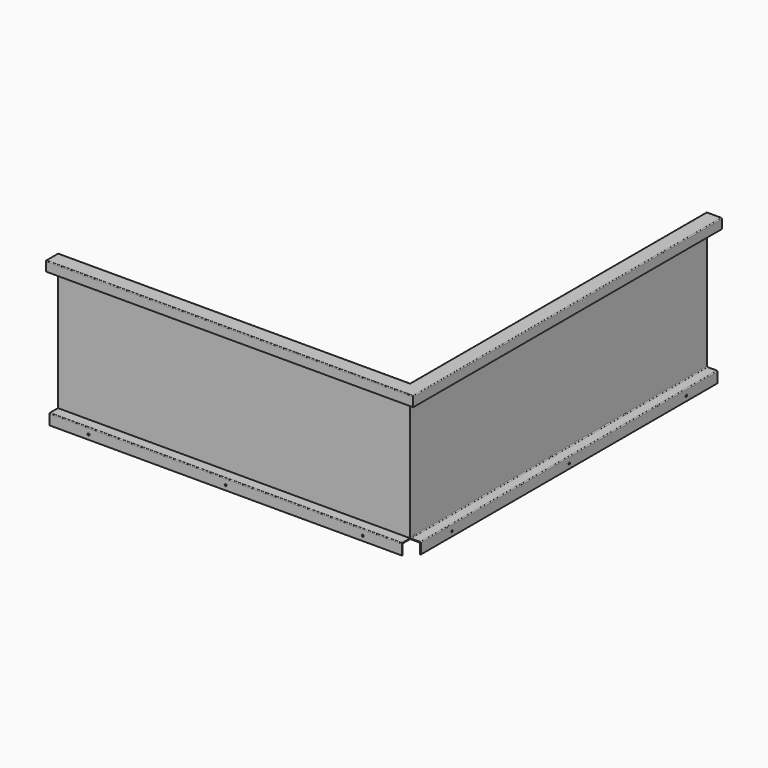
from build123d import *

# Parameters (mm, degrees)
F3_W         = 27
F3_H         = 27
F4_DEPTH     = 30
F5_T1_DEPTH  = 950
F5_T3_DEPTH  = 986
F5_T5_DEPTH  = 902
F5_T7_DEPTH  = 938
F5_T13_DEPTH = 955
F5_T17_DEPTH = 907
F5_T20_DEPTH = 960
F5_T22_DEPTH = 998
F5_T24_DEPTH = 953
F5_T26_DEPTH = 950
F5_T28_DEPTH = 905
F5_T30_DEPTH = 912
F5_T36_DEPTH = 910
F5_T40_DEPTH = 958
F5_T47_DEPTH = 910
F5_T51_DEPTH = 958
F8_D         = 5
F8_ON_F6_D   = 5


# Not quite as in the source:
# - a fillet or chamfer that OpenCascade refuses, or shapes differently, is made with other operations: its cross-section is extruded or revolved along the edge and cut away or added


with BuildPart() as f2:
    # F2: sweep along a path in F1
    with BuildLine(Plane.XY) as f2_path:
        Line((0, 0), (0, -948))
        Line((0, -948), (-900, -948))
    # F0 (on Front) → F2 (sweep)
    with BuildSketch(Plane.XZ):
        Polygon((38, -2), (38, -25), (40, -25), (40, 0), (0, 0), (0, -350), (27, -350), (27, -376), (29, -376), (29, -348), (2, -348), (2, -2), align=None)
    sweep(path=f2_path.line, transition=Transition.RIGHT)

    # F3 (on face) → F4 (cut)
    with BuildSketch(Plane.XY.offset(-348)):
        with Locations((15.5, -963.5)):
            Rectangle(F3_W, F3_H)
    extrude(amount=-F4_DEPTH, mode=Mode.SUBTRACT)

    # F5: fillet of radius 2 on 15 edges, made by hand

    # F5_s2 → F5_t1 (join)
    with BuildSketch(Plane.XZ):
        with BuildLine():
            ThreePointArc((2, -346), (2.5857864376, -347.4142135624), (4, -348))
            Line((4, -348), (2, -348))
            Line((2, -348), (2, -346))
        make_face()
        with BuildLine():
            ThreePointArc((25, -350), (26.4142135624, -350.5857864376), (27, -352))
            Line((27, -352), (27, -350))
            Line((27, -350), (25, -350))
        make_face()
        with BuildLine():
            ThreePointArc((4, -2), (2.5857864376, -2.5857864376), (2, -4))
            Line((2, -4), (2, -2))
            Line((2, -2), (4, -2))
        make_face()
    extrude(amount=F5_T1_DEPTH)

    # F5_s4 → F5_t3 (join)
    with BuildSketch(Plane.XZ):
        with BuildLine():
            ThreePointArc((38, -4), (37.4142135624, -2.5857864376), (36, -2))
            Line((36, -2), (38, -2))
            Line((38, -2), (38, -4))
        make_face()
    extrude(amount=F5_T3_DEPTH)

    # F5_s6 → F5_t5 (join)
    with BuildSketch(Plane.YZ.offset(-900)):
        with BuildLine():
            ThreePointArc((-973, -350), (-974.4142135624, -350.5857864376), (-975, -352))
            Line((-975, -352), (-975, -350))
            Line((-975, -350), (-973, -350))
        make_face()
        with BuildLine():
            ThreePointArc((-952, -2), (-950.5857864376, -2.5857864376), (-950, -4))
            Line((-950, -4), (-950, -2))
            Line((-950, -2), (-952, -2))
        make_face()
    extrude(amount=F5_T5_DEPTH)

    # F5_s8 → F5_t7 (join)
    with BuildSketch(Plane.YZ.offset(-900)):
        with BuildLine():
            ThreePointArc((-984, -2), (-985.4142135624, -2.5857864376), (-986, -4))
            Line((-986, -4), (-986, -2))
            Line((-986, -2), (-984, -2))
        make_face()
    extrude(amount=F5_T7_DEPTH)


with BuildPart() as f5_tool11:
    # F5_s12 → F5_t13 (new body)
    with BuildSketch(Plane.XZ):
        with BuildLine():
            ThreePointArc((4, -2), (2.5857864376, -2.5857864376), (2, -4))
            Line((2, -4), (2, -2))
            Line((2, -2), (4, -2))
        make_face()
    extrude(amount=F5_T13_DEPTH)

    split(bisect_by=Plane.XZ.offset(950), keep=Keep.TOP)


with BuildPart() as f5_tool15:
    # F5_s16 → F5_t17 (new body)
    with BuildSketch(Plane.YZ.offset(7)):
        with BuildLine():
            ThreePointArc((-952, -2), (-950.5857864376, -2.5857864376), (-950, -4))
            Line((-950, -4), (-950, -2))
            Line((-950, -2), (-952, -2))
        make_face()
    extrude(amount=-F5_T17_DEPTH)

    split(bisect_by=Plane.YZ.offset(2), keep=Keep.TOP)


with BuildPart() as f5_tool11_1:
    add(f5_tool11.part)

    # F5_t19: intersect F5_tool15
    add(f5_tool15.part, mode=Mode.INTERSECT)


with BuildPart() as f2_1:
    add(f2.part)

    # F5_t9: union F5_tool11
    add(f5_tool11_1.part)

    # F5_s21 → F5_t20 (cut)
    with BuildSketch(Plane.XZ.offset(-5)):
        with BuildLine():
            ThreePointArc((27, -348), (28.4142135624, -348.5857864376), (29, -350))
            Line((29, -350), (29, -348))
            Line((29, -348), (27, -348))
        make_face()
    extrude(amount=F5_T20_DEPTH, mode=Mode.SUBTRACT)

    # F5_s23 → F5_t22 (cut)
    with BuildSketch(Plane.XZ.offset(-5)):
        with BuildLine():
            ThreePointArc((38, 0), (39.4142135624, -0.5857864376), (40, -2))
            Line((40, -2), (40, 0))
            Line((40, 0), (38, 0))
        make_face()
    extrude(amount=F5_T22_DEPTH, mode=Mode.SUBTRACT)

    # F5_s25 → F5_t24 (cut)
    with BuildSketch(Plane.XZ.offset(-5)):
        with BuildLine():
            ThreePointArc((0, -2), (0.5857864376, -0.5857864376), (2, 0))
            Line((2, 0), (0, 0))
            Line((0, 0), (0, -2))
        make_face()
        with BuildLine():
            ThreePointArc((2, -350), (0.5857864376, -349.4142135624), (0, -348))
            Line((0, -348), (0, -350))
            Line((0, -350), (2, -350))
        make_face()
    extrude(amount=F5_T24_DEPTH, mode=Mode.SUBTRACT)

    # F5_s27 → F5_t26 (cut)
    with BuildSketch(Plane.YZ.offset(-905)):
        with BuildLine():
            ThreePointArc((-988, -2), (-987.4142135624, -0.5857864376), (-986, 0))
            Line((-986, 0), (-988, 0))
            Line((-988, 0), (-988, -2))
        make_face()
    extrude(amount=F5_T26_DEPTH, mode=Mode.SUBTRACT)

    # F5_s29 → F5_t28 (cut)
    with BuildSketch(Plane.YZ.offset(-905)):
        with BuildLine():
            ThreePointArc((-948, -2), (-948.5857864376, -0.5857864376), (-950, 0))
            Line((-950, 0), (-948, 0))
            Line((-948, 0), (-948, -2))
        make_face()
        with BuildLine():
            ThreePointArc((-948, -348), (-948.5857864376, -349.4142135624), (-950, -350))
            Line((-950, -350), (-948, -350))
            Line((-948, -350), (-948, -348))
        make_face()
    extrude(amount=F5_T28_DEPTH, mode=Mode.SUBTRACT)

    # F5_s31 → F5_t30 (cut)
    with BuildSketch(Plane.YZ.offset(-905)):
        with BuildLine():
            ThreePointArc((-977, -350), (-976.4142135624, -348.5857864376), (-975, -348))
            Line((-975, -348), (-977, -348))
            Line((-977, -348), (-977, -350))
        make_face()
    extrude(amount=F5_T30_DEPTH, mode=Mode.SUBTRACT)


with BuildPart() as f5_tool34:
    # F5_s35 → F5_t36 (new body)
    with BuildSketch(Plane.YZ.offset(5)):
        with BuildLine():
            ThreePointArc((-948, -2), (-948.5857864376, -0.5857864376), (-950, 0))
            Line((-950, 0), (-948, 0))
            Line((-948, 0), (-948, -2))
        make_face()
    extrude(amount=-F5_T36_DEPTH)

    split(bisect_by=Plane.YZ, keep=Keep.TOP)


with BuildPart() as f5_tool38:
    # F5_s39 → F5_t40 (new body)
    with BuildSketch(Plane.XZ.offset(-5)):
        with BuildLine():
            ThreePointArc((0, -2), (0.5857864376, -0.5857864376), (2, 0))
            Line((2, 0), (0, 0))
            Line((0, 0), (0, -2))
        make_face()
    extrude(amount=F5_T40_DEPTH)

    split(bisect_by=Plane.XZ.offset(948), keep=Keep.TOP)


with BuildPart() as f5_tool34_1:
    add(f5_tool34.part)

    # F5_t42: intersect F5_tool38
    add(f5_tool38.part, mode=Mode.INTERSECT)


with BuildPart() as f2_2:
    add(f2_1.part)

    # F5_t32: cut F5_tool34
    add(f5_tool34_1.part, mode=Mode.SUBTRACT)


with BuildPart() as f5_tool45:
    # F5_s46 → F5_t47 (new body)
    with BuildSketch(Plane.YZ.offset(5)):
        with BuildLine():
            ThreePointArc((-948, -348), (-948.5857864376, -349.4142135624), (-950, -350))
            Line((-950, -350), (-948, -350))
            Line((-948, -350), (-948, -348))
        make_face()
    extrude(amount=-F5_T47_DEPTH)

    split(bisect_by=Plane.YZ, keep=Keep.TOP)


with BuildPart() as f5_tool49:
    # F5_s50 → F5_t51 (new body)
    with BuildSketch(Plane.XZ.offset(-5)):
        with BuildLine():
            ThreePointArc((2, -350), (0.5857864376, -349.4142135624), (0, -348))
            Line((0, -348), (0, -350))
            Line((0, -350), (2, -350))
        make_face()
    extrude(amount=F5_T51_DEPTH)

    split(bisect_by=Plane.XZ.offset(948), keep=Keep.TOP)


with BuildPart() as f5_tool45_1:
    add(f5_tool45.part)

    # F5_t53: intersect F5_tool49
    add(f5_tool49.part, mode=Mode.INTERSECT)


with BuildPart() as f2_3:
    add(f2_2.part)

    # F5_t43: cut F5_tool45
    add(f5_tool45_1.part, mode=Mode.SUBTRACT)

    # F8 (through all)
    with Locations(Plane(origin=(0, -975, 0), x_dir=(-1, 0, 0), z_dir=(0, 1, 0))):
        with Locations((98, -364), (449, -364), (800, -364)):
            Hole(F8_D / 2)

    # F8 on F6 (through all)
    with Locations(Plane(origin=(27, 0, 0), x_dir=(0, -1, 0), z_dir=(-1, 0, 0))):
        with Locations((100, -364), (475, -364), (850, -364)):
            Hole(F8_ON_F6_D / 2)


solid = f2_3.part
